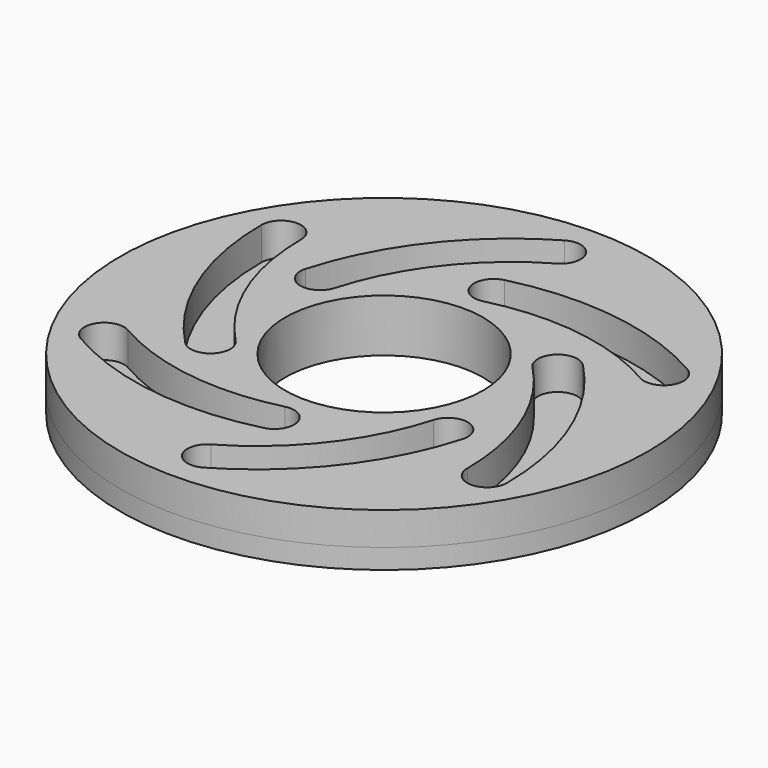
from build123d import *

# Parameters (mm, degrees)
F0_R     = 40
F0_R_2   = 15
F1_DEPTH = 8
F2_R     = 40
F2_R_2   = 1.75
F2_R_3   = 16.5
F3_DEPTH = 3


with BuildPart() as f1:
    # F0 (on Top) → F1 (new body)
    with BuildSketch(Plane.XY):
        Circle(F0_R)
        with BuildLine():
            ThreePointArc((0.732503888, -23.6938085589), (-15.3080829926, -24.5623956339), (-30.5, -19.3412340179))
            ThreePointArc((-30.5, -19.3412340179), (-31.5980762114, -15.2431578065), (-27.5, -14.1450815951))
            ThreePointArc((-27.5, -14.1450815951), (-14.4799238355, -18.6198244386), (-0.732503888, -17.8754108227))
            ThreePointArc((-0.732503888, -17.8754108227), (2.9091988681, -20.0521058028), (0.732503888, -23.6938085589))
        make_face(mode=Mode.SUBTRACT)
        with BuildLine():
            ThreePointArc((20.8856920684, -11.2125373041), (13.6176171004, -25.5383865717), (1.5, -36.0843918244))
            ThreePointArc((1.5, -36.0843918244), (-2.5980762114, -34.986315613), (-1.5, -30.8882394016))
            ThreePointArc((-1.5, -30.8882394016), (8.8852790601, -21.8498941057), (15.1143079316, -9.5720723868))
            ThreePointArc((15.1143079316, -9.5720723868), (18.8202324586, -7.506612777), (20.8856920684, -11.2125373041))
        make_face(mode=Mode.SUBTRACT)
        with BuildLine():
            ThreePointArc((20.1531881804, 12.4812712549), (28.925700093, -0.9759909379), (32, -16.7431578065))
            ThreePointArc((32, -16.7431578065), (29, -19.7431578065), (26, -16.7431578065))
            ThreePointArc((26, -16.7431578065), (23.3652028956, -3.2300696671), (15.8468118196, 8.303338436))
            ThreePointArc((15.8468118196, 8.303338436), (15.9110335906, 12.5454930258), (20.1531881804, 12.4812712549))
        make_face(mode=Mode.SUBTRACT)
        with BuildLine():
            ThreePointArc((-20.1531881804, -12.4812712549), (-28.925700093, 0.9759909379), (-32, 16.7431578065))
            ThreePointArc((-32, 16.7431578065), (-29, 19.7431578065), (-26, 16.7431578065))
            ThreePointArc((-26, 16.7431578065), (-23.3652028956, 3.2300696671), (-15.8468118196, -8.303338436))
            ThreePointArc((-15.8468118196, -8.303338436), (-15.9110335906, -12.5454930258), (-20.1531881804, -12.4812712549))
        make_face(mode=Mode.SUBTRACT)
        with BuildLine():
            ThreePointArc((-20.8856920684, 11.2125373041), (-13.6176171004, 25.5383865717), (-1.5, 36.0843918244))
            ThreePointArc((-1.5, 36.0843918244), (2.5980762114, 34.986315613), (1.5, 30.8882394016))
            ThreePointArc((1.5, 30.8882394016), (-8.8852790601, 21.8498941057), (-15.1143079316, 9.5720723868))
            ThreePointArc((-15.1143079316, 9.5720723868), (-18.8202324586, 7.506612777), (-20.8856920684, 11.2125373041))
        make_face(mode=Mode.SUBTRACT)
        Circle(F0_R_2, mode=Mode.SUBTRACT)
        with BuildLine():
            ThreePointArc((-0.732503888, 23.6938085589), (15.3080829926, 24.5623956339), (30.5, 19.3412340179))
            ThreePointArc((30.5, 19.3412340179), (31.5980762114, 15.2431578065), (27.5, 14.1450815951))
            ThreePointArc((27.5, 14.1450815951), (14.4799238355, 18.6198244386), (0.732503888, 17.8754108227))
            ThreePointArc((0.732503888, 17.8754108227), (-2.9091988681, 20.0521058028), (-0.732503888, 23.6938085589))
        make_face(mode=Mode.SUBTRACT)
    extrude(amount=F1_DEPTH)


with BuildPart() as f3:
    # F2 (on Top) → F3 (new body)
    with BuildSketch(Plane.XY):
        Circle(F2_R)
        with Locations((18, -31.1769145362)):
            Circle(F2_R_2, mode=Mode.SUBTRACT)
        with Locations((-36, 0)):
            Circle(F2_R_2, mode=Mode.SUBTRACT)
        Circle(F2_R_3, mode=Mode.SUBTRACT)
        with Locations((18, 31.1769145362)):
            Circle(F2_R_2, mode=Mode.SUBTRACT)
    extrude(amount=F3_DEPTH)


solid = Compound([f1.part, f3.part])
